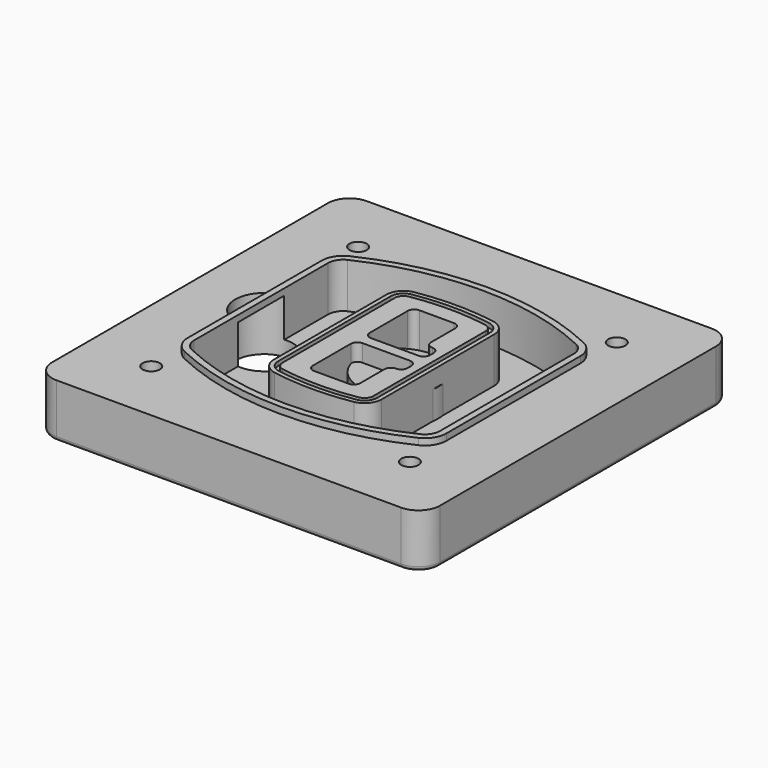
from build123d import *

# Parameters (mm, degrees)
F0_R      = 4
F1_DEPTH  = 25
F2_DEPTH  = 3
F3_DEPTH  = 18
F5_DEPTH  = 21
F6_DEPTH  = 2
F8_DEPTH  = 20
F9_DEPTH  = 16
F10_DEPTH = 25
F7_R      = 6
F7_R_2    = 4
F11_DEPTH = 6
F13_DEPTH = 9
F15_R     = 2


# Not quite as in the source:
# - a feature of the source that left no trace in its solid (it failed there, or was rolled back) is left out
# - a feature names something its author has since deleted; it is built from what else it names


with BuildPart() as f1:
    # F0 (on Top) → F1 (new body)
    with BuildSketch(Plane.XY):
        with BuildLine():
            ThreePointArc((-90, -80), (-87.0710678119, -87.0710678119), (-80, -90))
            Line((-80, -90), (80, -90))
            ThreePointArc((80, -90), (87.0710678119, -87.0710678119), (90, -80))
            Line((90, -80), (90, 80))
            ThreePointArc((90, 80), (87.0710678119, 87.0710678119), (80, 90))
            Line((80, 90), (-80, 90))
            ThreePointArc((-80, 90), (-87.0710678119, 87.0710678119), (-90, 80))
            Line((-90, 80), (-90, -80))
        make_face()
        with Locations((-60, -60)):
            Circle(F0_R, mode=Mode.SUBTRACT)
        with Locations((60, -60)):
            Circle(F0_R, mode=Mode.SUBTRACT)
        with Locations((-60, 60)):
            Circle(F0_R, mode=Mode.SUBTRACT)
        with BuildLine():
            ThreePointArc((-64, 38.8308515907), (-61.8195654598, 46.3340424013), (-55.9574468085, 51.5000594398))
            ThreePointArc((-55.9574468085, 51.5000594398), (0, 64), (55.9574468085, 51.5000594398))
            ThreePointArc((55.9574468085, 51.5000594398), (61.8195654598, 46.3340424013), (64, 38.8308515907))
            Line((64, 38.8308515907), (64, -38.8308515907))
            ThreePointArc((64, -38.8308515907), (61.8195654598, -46.3340424013), (55.9574468085, -51.5000594398))
            ThreePointArc((55.9574468085, -51.5000594398), (0, -64), (-55.9574468085, -51.5000594398))
            ThreePointArc((-55.9574468085, -51.5000594398), (-61.8195654598, -46.3340424013), (-64, -38.8308515907))
            Line((-64, -38.8308515907), (-64, 38.8308515907))
        make_face(mode=Mode.SUBTRACT)
        with Locations((60, 60)):
            Circle(F0_R, mode=Mode.SUBTRACT)
        with BuildLine():
            ThreePointArc((55.9574468085, 51.5000594398), (0, 64), (-55.9574468085, 51.5000594398))
            ThreePointArc((-55.9574468085, 51.5000594398), (-61.8195654598, 46.3340424013), (-64, 38.8308515907))
            Line((-64, 38.8308515907), (-64, -38.8308515907))
            ThreePointArc((-64, -38.8308515907), (-61.8195654598, -46.3340424013), (-55.9574468085, -51.5000594398))
            ThreePointArc((-55.9574468085, -51.5000594398), (0, -64), (55.9574468085, -51.5000594398))
            ThreePointArc((55.9574468085, -51.5000594398), (61.8195654598, -46.3340424013), (64, -38.8308515907))
            Line((64, -38.8308515907), (64, 38.8308515907))
            ThreePointArc((64, 38.8308515907), (61.8195654598, 46.3340424013), (55.9574468085, 51.5000594398))
        make_face()
        with BuildLine():
            Line((-60, -38.8308515907), (-60, 38.8308515907))
            ThreePointArc((-60, 38.8308515907), (-58.442546757, 44.1902735983), (-54.2553191489, 47.8802857686))
            ThreePointArc((-54.2553191489, 47.8802857686), (0, 60), (54.2553191489, 47.8802857686))
            ThreePointArc((54.2553191489, 47.8802857686), (58.442546757, 44.1902735983), (60, 38.8308515907))
            Line((60, 38.8308515907), (60, -38.8308515907))
            ThreePointArc((60, -38.8308515907), (58.442546757, -44.1902735983), (54.2553191489, -47.8802857686))
            ThreePointArc((54.2553191489, -47.8802857686), (0, -60), (-54.2553191489, -47.8802857686))
            ThreePointArc((-54.2553191489, -47.8802857686), (-58.442546757, -44.1902735983), (-60, -38.8308515907))
        make_face(mode=Mode.SUBTRACT)
        with BuildLine():
            ThreePointArc((-54.2553191489, 47.8802857686), (-58.442546757, 44.1902735983), (-60, 38.8308515907))
            Line((-60, 38.8308515907), (-60, -38.8308515907))
            ThreePointArc((-60, -38.8308515907), (-58.442546757, -44.1902735983), (-54.2553191489, -47.8802857686))
            ThreePointArc((-54.2553191489, -47.8802857686), (0, -60), (54.2553191489, -47.8802857686))
            ThreePointArc((54.2553191489, -47.8802857686), (58.442546757, -44.1902735983), (60, -38.8308515907))
            Line((60, -38.8308515907), (60, 38.8308515907))
            ThreePointArc((60, 38.8308515907), (58.442546757, 44.1902735983), (54.2553191489, 47.8802857686))
            ThreePointArc((54.2553191489, 47.8802857686), (0, 60), (-54.2553191489, 47.8802857686))
        make_face()
        with BuildLine():
            ThreePointArc((52.9787234043, 45.1654555152), (55.9097827299, 42.582446996), (57, 38.8308515907))
            Line((57, 38.8308515907), (57, -38.8308515907))
            ThreePointArc((57, -38.8308515907), (55.9097827299, -42.582446996), (52.9787234043, -45.1654555152))
            ThreePointArc((52.9787234043, -45.1654555152), (0, -57), (-52.9787234043, -45.1654555152))
            ThreePointArc((-52.9787234043, -45.1654555152), (-55.9097827299, -42.582446996), (-57, -38.8308515907))
            Line((-57, -38.8308515907), (-57, 38.8308515907))
            ThreePointArc((-57, 38.8308515907), (-55.9097827299, 42.582446996), (-52.9787234043, 45.1654555152))
            ThreePointArc((-52.9787234043, 45.1654555152), (0, 57), (52.9787234043, 45.1654555152))
        make_face(mode=Mode.SUBTRACT)
        with BuildLine():
            Line((57, -38.8308515907), (57, 38.8308515907))
            ThreePointArc((57, 38.8308515907), (55.9097827299, 42.582446996), (52.9787234043, 45.1654555152))
            ThreePointArc((52.9787234043, 45.1654555152), (0, 57), (-52.9787234043, 45.1654555152))
            ThreePointArc((-52.9787234043, 45.1654555152), (-55.9097827299, 42.582446996), (-57, 38.8308515907))
            Line((-57, 38.8308515907), (-57, -38.8308515907))
            ThreePointArc((-57, -38.8308515907), (-55.9097827299, -42.582446996), (-52.9787234043, -45.1654555152))
            ThreePointArc((-52.9787234043, -45.1654555152), (0, -57), (52.9787234043, -45.1654555152))
            ThreePointArc((52.9787234043, -45.1654555152), (55.9097827299, -42.582446996), (57, -38.8308515907))
        make_face()
    extrude(amount=-F1_DEPTH)

    # F0 (on Top) → F2 (join)
    with BuildSketch(Plane.XY):
        with BuildLine():
            ThreePointArc((-54.2553191489, 47.8802857686), (-58.442546757, 44.1902735983), (-60, 38.8308515907))
            Line((-60, 38.8308515907), (-60, -38.8308515907))
            ThreePointArc((-60, -38.8308515907), (-58.442546757, -44.1902735983), (-54.2553191489, -47.8802857686))
            ThreePointArc((-54.2553191489, -47.8802857686), (0, -60), (54.2553191489, -47.8802857686))
            ThreePointArc((54.2553191489, -47.8802857686), (58.442546757, -44.1902735983), (60, -38.8308515907))
            Line((60, -38.8308515907), (60, 38.8308515907))
            ThreePointArc((60, 38.8308515907), (58.442546757, 44.1902735983), (54.2553191489, 47.8802857686))
            ThreePointArc((54.2553191489, 47.8802857686), (0, 60), (-54.2553191489, 47.8802857686))
        make_face()
        with BuildLine():
            ThreePointArc((52.9787234043, 45.1654555152), (55.9097827299, 42.582446996), (57, 38.8308515907))
            Line((57, 38.8308515907), (57, -38.8308515907))
            ThreePointArc((57, -38.8308515907), (55.9097827299, -42.582446996), (52.9787234043, -45.1654555152))
            ThreePointArc((52.9787234043, -45.1654555152), (0, -57), (-52.9787234043, -45.1654555152))
            ThreePointArc((-52.9787234043, -45.1654555152), (-55.9097827299, -42.582446996), (-57, -38.8308515907))
            Line((-57, -38.8308515907), (-57, 38.8308515907))
            ThreePointArc((-57, 38.8308515907), (-55.9097827299, 42.582446996), (-52.9787234043, 45.1654555152))
            ThreePointArc((-52.9787234043, 45.1654555152), (0, 57), (52.9787234043, 45.1654555152))
        make_face(mode=Mode.SUBTRACT)
    extrude(amount=F2_DEPTH)

    # F0 (on Top) → F3 (cut)
    with BuildSketch(Plane.XY):
        with BuildLine():
            Line((57, -38.8308515907), (57, 38.8308515907))
            ThreePointArc((57, 38.8308515907), (55.9097827299, 42.582446996), (52.9787234043, 45.1654555152))
            ThreePointArc((52.9787234043, 45.1654555152), (0, 57), (-52.9787234043, 45.1654555152))
            ThreePointArc((-52.9787234043, 45.1654555152), (-55.9097827299, 42.582446996), (-57, 38.8308515907))
            Line((-57, 38.8308515907), (-57, -38.8308515907))
            ThreePointArc((-57, -38.8308515907), (-55.9097827299, -42.582446996), (-52.9787234043, -45.1654555152))
            ThreePointArc((-52.9787234043, -45.1654555152), (0, -57), (52.9787234043, -45.1654555152))
            ThreePointArc((52.9787234043, -45.1654555152), (55.9097827299, -42.582446996), (57, -38.8308515907))
        make_face()
    extrude(amount=-F3_DEPTH, mode=Mode.SUBTRACT)

    # F4 (on face) → F5 (join, through all)
    with BuildSketch(Plane.XY.offset(3)):
        with BuildLine():
            ThreePointArc((-25, -32.5662280692), (-23.1122504785, -37.7276614059), (-18.3399014778, -40.4532214146))
            ThreePointArc((-18.3399014778, -40.4532214146), (0, -42), (18.3399014778, -40.4532214146))
            ThreePointArc((18.3399014778, -40.4532214146), (23.1122504785, -37.7276614059), (25, -32.5662280692))
            Line((25, -32.5662280692), (25, 32.5662280692))
            ThreePointArc((25, 32.5662280692), (23.1122504785, 37.7276614059), (18.3399014778, 40.4532214146))
            ThreePointArc((18.3399014778, 40.4532214146), (0, 42), (-18.3399014778, 40.4532214146))
            ThreePointArc((-18.3399014778, 40.4532214146), (-23.1122504785, 37.7276614059), (-25, 32.5662280692))
            Line((-25, 32.5662280692), (-25, -32.5662280692))
        make_face()
        with BuildLine():
            ThreePointArc((18.0049261084, 38.4814730782), (21.5841878588, 36.4373030717), (23, 32.5662280692))
            Line((23, 32.5662280692), (23, -32.5662280692))
            ThreePointArc((23, -32.5662280692), (21.5841878588, -36.4373030717), (18.0049261084, -38.4814730782))
            ThreePointArc((18.0049261084, -38.4814730782), (0, -40), (-18.0049261084, -38.4814730782))
            ThreePointArc((-18.0049261084, -38.4814730782), (-21.5841878588, -36.4373030717), (-23, -32.5662280692))
            Line((-23, -32.5662280692), (-23, 32.5662280692))
            ThreePointArc((-23, 32.5662280692), (-21.5841878588, 36.4373030717), (-18.0049261084, 38.4814730782))
            ThreePointArc((-18.0049261084, 38.4814730782), (0, 40), (18.0049261084, 38.4814730782))
        make_face(mode=Mode.SUBTRACT)
        with BuildLine():
            Line((23, -32.5662280692), (23, 32.5662280692))
            ThreePointArc((23, 32.5662280692), (21.5841878588, 36.4373030717), (18.0049261084, 38.4814730782))
            ThreePointArc((18.0049261084, 38.4814730782), (0, 40), (-18.0049261084, 38.4814730782))
            ThreePointArc((-18.0049261084, 38.4814730782), (-21.5841878588, 36.4373030717), (-23, 32.5662280692))
            Line((-23, 32.5662280692), (-23, -32.5662280692))
            ThreePointArc((-23, -32.5662280692), (-21.5841878588, -36.4373030717), (-18.0049261084, -38.4814730782))
            ThreePointArc((-18.0049261084, -38.4814730782), (0, -40), (18.0049261084, -38.4814730782))
            ThreePointArc((18.0049261084, -38.4814730782), (21.5841878588, -36.4373030717), (23, -32.5662280692))
        make_face()
        with BuildLine():
            ThreePointArc((17.6699507389, 36.5097247419), (20.0561252392, 35.1469447375), (21, 32.5662280692))
            Line((21, 32.5662280692), (21, -32.5662280692))
            ThreePointArc((21, -32.5662280692), (20.0561252392, -35.1469447375), (17.6699507389, -36.5097247419))
            ThreePointArc((17.6699507389, -36.5097247419), (0, -38), (-17.6699507389, -36.5097247419))
            ThreePointArc((-17.6699507389, -36.5097247419), (-20.0561252392, -35.1469447375), (-21, -32.5662280692))
            Line((-21, -32.5662280692), (-21, 32.5662280692))
            ThreePointArc((-21, 32.5662280692), (-20.0561252392, 35.1469447375), (-17.6699507389, 36.5097247419))
            ThreePointArc((-17.6699507389, 36.5097247419), (0, 38), (17.6699507389, 36.5097247419))
        make_face(mode=Mode.SUBTRACT)
        with BuildLine():
            Line((21, -32.5662280692), (21, 32.5662280692))
            ThreePointArc((21, 32.5662280692), (20.0561252392, 35.1469447375), (17.6699507389, 36.5097247419))
            ThreePointArc((17.6699507389, 36.5097247419), (0, 38), (-17.6699507389, 36.5097247419))
            ThreePointArc((-17.6699507389, 36.5097247419), (-20.0561252392, 35.1469447375), (-21, 32.5662280692))
            Line((-21, 32.5662280692), (-21, -32.5662280692))
            ThreePointArc((-21, -32.5662280692), (-20.0561252392, -35.1469447375), (-17.6699507389, -36.5097247419))
            ThreePointArc((-17.6699507389, -36.5097247419), (0, -38), (17.6699507389, -36.5097247419))
            ThreePointArc((17.6699507389, -36.5097247419), (20.0561252392, -35.1469447375), (21, -32.5662280692))
        make_face()
        with BuildLine():
            Line((-8, -2.5), (14, -2.5))
            ThreePointArc((14, -2.5), (16.1213203436, -3.3786796564), (17, -5.5))
            Line((17, -5.5), (17, -7.5))
            ThreePointArc((17, -7.5), (16.1213203436, -9.6213203436), (14, -10.5))
            ThreePointArc((14, -10.5), (11.8786796564, -11.3786796564), (11, -13.5))
            Line((11, -13.5), (11, -27.5))
            ThreePointArc((11, -27.5), (10.1213203436, -29.6213203436), (8, -30.5))
            Line((8, -30.5), (-8, -30.5))
            ThreePointArc((-8, -30.5), (-10.1213203436, -29.6213203436), (-11, -27.5))
            Line((-11, -27.5), (-11, -5.5))
            ThreePointArc((-11, -5.5), (-10.1213203436, -3.3786796564), (-8, -2.5))
        make_face(mode=Mode.SUBTRACT)
        with BuildLine():
            ThreePointArc((-8, 2.5), (-10.1213203436, 3.3786796564), (-11, 5.5))
            Line((-11, 5.5), (-11, 27.5))
            ThreePointArc((-11, 27.5), (-10.1213203436, 29.6213203436), (-8, 30.5))
            Line((-8, 30.5), (8, 30.5))
            ThreePointArc((8, 30.5), (10.1213203436, 29.6213203436), (11, 27.5))
            Line((11, 27.5), (11, 13.5))
            ThreePointArc((11, 13.5), (11.8786796564, 11.3786796564), (14, 10.5))
            ThreePointArc((14, 10.5), (16.1213203436, 9.6213203436), (17, 7.5))
            Line((17, 7.5), (17, 5.5))
            ThreePointArc((17, 5.5), (16.1213203436, 3.3786796564), (14, 2.5))
            Line((14, 2.5), (-8, 2.5))
        make_face(mode=Mode.SUBTRACT)
    extrude(amount=-F5_DEPTH)

    # F4 (on face) → F6 (cut)
    with BuildSketch(Plane.XY.offset(3)):
        with BuildLine():
            Line((23, -32.5662280692), (23, 32.5662280692))
            ThreePointArc((23, 32.5662280692), (21.5841878588, 36.4373030717), (18.0049261084, 38.4814730782))
            ThreePointArc((18.0049261084, 38.4814730782), (0, 40), (-18.0049261084, 38.4814730782))
            ThreePointArc((-18.0049261084, 38.4814730782), (-21.5841878588, 36.4373030717), (-23, 32.5662280692))
            Line((-23, 32.5662280692), (-23, -32.5662280692))
            ThreePointArc((-23, -32.5662280692), (-21.5841878588, -36.4373030717), (-18.0049261084, -38.4814730782))
            ThreePointArc((-18.0049261084, -38.4814730782), (0, -40), (18.0049261084, -38.4814730782))
            ThreePointArc((18.0049261084, -38.4814730782), (21.5841878588, -36.4373030717), (23, -32.5662280692))
        make_face()
        with BuildLine():
            ThreePointArc((17.6699507389, 36.5097247419), (20.0561252392, 35.1469447375), (21, 32.5662280692))
            Line((21, 32.5662280692), (21, -32.5662280692))
            ThreePointArc((21, -32.5662280692), (20.0561252392, -35.1469447375), (17.6699507389, -36.5097247419))
            ThreePointArc((17.6699507389, -36.5097247419), (0, -38), (-17.6699507389, -36.5097247419))
            ThreePointArc((-17.6699507389, -36.5097247419), (-20.0561252392, -35.1469447375), (-21, -32.5662280692))
            Line((-21, -32.5662280692), (-21, 32.5662280692))
            ThreePointArc((-21, 32.5662280692), (-20.0561252392, 35.1469447375), (-17.6699507389, 36.5097247419))
            ThreePointArc((-17.6699507389, 36.5097247419), (0, 38), (17.6699507389, 36.5097247419))
        make_face(mode=Mode.SUBTRACT)
    extrude(amount=-F6_DEPTH, mode=Mode.SUBTRACT)

    # F7 (on face) → F8 (join)
    with BuildSketch(Plane(origin=(0, 0, -25), x_dir=(1, 0, 0), z_dir=(0, 0, -1))):
        with BuildLine():
            ThreePointArc((-6.71157564, 0), (6.7567035675, 13.4682792075), (20.224982775, 0))
            Line((20.224982775, 0), (25.224982775, 0))
            ThreePointArc((25.224982775, 0), (6.7567035675, 18.4682792075), (-11.71157564, 0))
            Line((-11.71157564, 0), (-6.71157564, 0))
        make_face()
        with BuildLine():
            Line((-6.71157564, 0), (20.224982775, 0))
            ThreePointArc((20.224982775, 0), (6.7567035675, 13.4682792075), (-6.71157564, 0))
        make_face()
        with BuildLine():
            ThreePointArc((-6.71157564, 0), (6.7567035675, -13.4682792075), (20.224982775, 0))
            Line((20.224982775, 0), (-6.71157564, 0))
        make_face()
        with BuildLine():
            Line((25.224982775, 0), (20.224982775, 0))
            ThreePointArc((20.224982775, 0), (6.7567035675, -13.4682792075), (-6.71157564, 0))
            Line((-6.71157564, 0), (-11.71157564, 0))
            ThreePointArc((-11.71157564, 0), (6.7567035675, -18.4682792075), (25.224982775, 0))
        make_face()
    extrude(amount=-F8_DEPTH)

    # F7 (on face) → F9 (cut)
    with BuildSketch(Plane(origin=(0, 0, -25), x_dir=(1, 0, 0), z_dir=(0, 0, -1))):
        with BuildLine():
            Line((-6.71157564, 0), (20.224982775, 0))
            ThreePointArc((20.224982775, 0), (6.7567035675, 13.4682792075), (-6.71157564, 0))
        make_face()
        with BuildLine():
            ThreePointArc((-6.71157564, 0), (6.7567035675, -13.4682792075), (20.224982775, 0))
            Line((20.224982775, 0), (-6.71157564, 0))
        make_face()
    extrude(amount=-F9_DEPTH, mode=Mode.SUBTRACT)

    # F7 (on face) → F10 (cut)
    with BuildSketch(Plane(origin=(0, 0, -25), x_dir=(1, 0, 0), z_dir=(0, 0, -1))):
        with BuildLine():
            Line((-69.0318229325, 0), (-42.0952645175, 0))
            ThreePointArc((-42.0952645175, 0), (-55.563543725, 13.4682792075), (-69.0318229325, 0))
        make_face()
        with BuildLine():
            ThreePointArc((-69.0318229325, 0), (-55.563543725, -13.4682792075), (-42.0952645175, 0))
            Line((-42.0952645175, 0), (-69.0318229325, 0))
        make_face()
    extrude(amount=-F10_DEPTH, mode=Mode.SUBTRACT)

    # F7 (on face) → F11 (cut)
    with BuildSketch(Plane(origin=(0, 0, -25), x_dir=(1, 0, 0), z_dir=(0, 0, -1))):
        with Locations((60, -60)):
            Circle(F7_R)
        with Locations((60, -60)):
            Circle(F7_R_2, mode=Mode.SUBTRACT)
        with Locations((-60, -60)):
            Circle(F7_R)
        with Locations((-60, -60)):
            Circle(F7_R_2, mode=Mode.SUBTRACT)
        with Locations((-60, 60)):
            Circle(F7_R)
        with Locations((-60, 60)):
            Circle(F7_R_2, mode=Mode.SUBTRACT)
        with Locations((60, 60)):
            Circle(F7_R)
        with Locations((60, 60)):
            Circle(F7_R_2, mode=Mode.SUBTRACT)
    extrude(amount=-F11_DEPTH, mode=Mode.SUBTRACT)

    # F12 (on face) → F13 (cut, through all)
    with BuildSketch(Plane(origin=(0, 0, -9), x_dir=(1, 0, 0), z_dir=(0, 0, -1))):
        with BuildLine():
            ThreePointArc((20.224982775, 0), (20.1663399806, 1.2554664788), (19.9909222755, 2.5))
            Line((19.9909222755, 2.5), (14, 2.5))
            ThreePointArc((14, 2.5), (16.1213203436, 3.3786796564), (17, 5.5))
            Line((17, 5.5), (17, 7.5))
            ThreePointArc((17, 7.5), (16.1213203436, 9.6213203436), (14, 10.5))
            ThreePointArc((14, 10.5), (12.1627255951, 11.1284134507), (11.0951631559, 12.750384826))
            ThreePointArc((11.0951631559, 12.750384826), (11.0476113807, 12.7664660322), (11, 12.7823698976))
            Line((11, 12.7823698976), (11, -12.7823698976))
            ThreePointArc((11, -12.7823698976), (11.0476113807, -12.7664660322), (11.0951631559, -12.750384826))
            ThreePointArc((11.0951631559, -12.750384826), (12.1627255951, -11.1284134507), (14, -10.5))
            ThreePointArc((14, -10.5), (16.1213203436, -9.6213203436), (17, -7.5))
            Line((17, -7.5), (17, -5.5))
            ThreePointArc((17, -5.5), (16.1213203436, -3.3786796564), (14, -2.5))
            Line((14, -2.5), (19.9909222755, -2.5))
            ThreePointArc((19.9909222755, -2.5), (20.1663399806, -1.2554664788), (20.224982775, 0))
        make_face()
    extrude(amount=F13_DEPTH, mode=Mode.SUBTRACT)

    # F15
    f15_edges = [f1.edges().sort_by_distance(p)[0] for p in [
        (0, -90, -25),
        (-87.071068, -87.071068, -25),
        (-90, 0, -25),
        (-87.071068, 87.071068, -25),
        (87.071068, -87.071068, -25),
        (0, 90, -25),
        (90, 0, -25),
        (87.071068, 87.071068, -25),
    ]]
    fillet(f15_edges, radius=F15_R)


solid = f1.part
